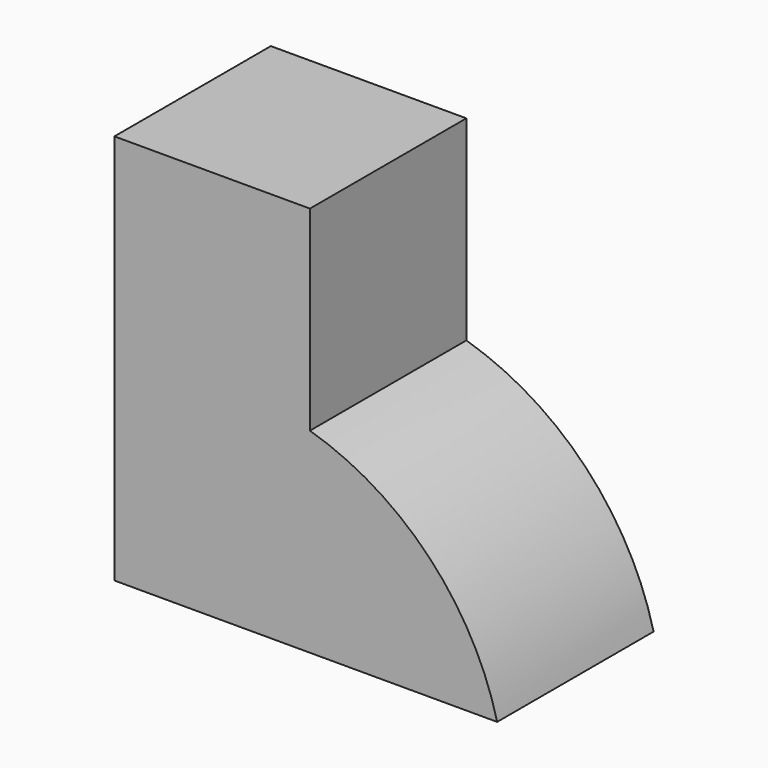
from build123d import *

# Parameters (mm, degrees)
F1_DEPTH    = 25.4
F2_T1_DEPTH = 195.8114627457


# Not quite as in the source:
# - a fillet or chamfer that OpenCascade refuses, or shapes differently, is made with other operations: its cross-section is extruded or revolved along the edge and cut away or added


with BuildPart() as f1:
    # F0 (on Front) → F1 (new body)
    with BuildSketch(Plane.XZ):
        Polygon((0, 50.8), (0, 0), (50.8, 0), (50.8, 25.4), (25.4, 25.4), (25.4, 50.8), align=None)
    extrude(amount=F1_DEPTH)

    # F2: fillet of radius 35.5661942009 on 1 edges, made by hand

    # F2_s2 → F2_t1 (cut)
    with BuildSketch(Plane.XZ.offset(-85.2057313728)):
        with BuildLine():
            ThreePointArc((50.8, -8.6822925491), (43.7515810206, 12.5707229158), (25.4, 25.4))
            Line((25.4, 25.4), (25.603323884, 26.081645851))
            ThreePointArc((25.603323884, 26.081645851), (38.1, 26.111323884), (50.8, 26.111323884))
            Line((50.8, 26.111323884), (51.511323884, 25.4))
            Line((51.511323884, 25.4), (51.511323884, -8.6822925491))
            Line((51.511323884, -8.6822925491), (50.8, -8.6822925491))
        make_face()
    extrude(amount=F2_T1_DEPTH, mode=Mode.SUBTRACT)


solid = f1.part
